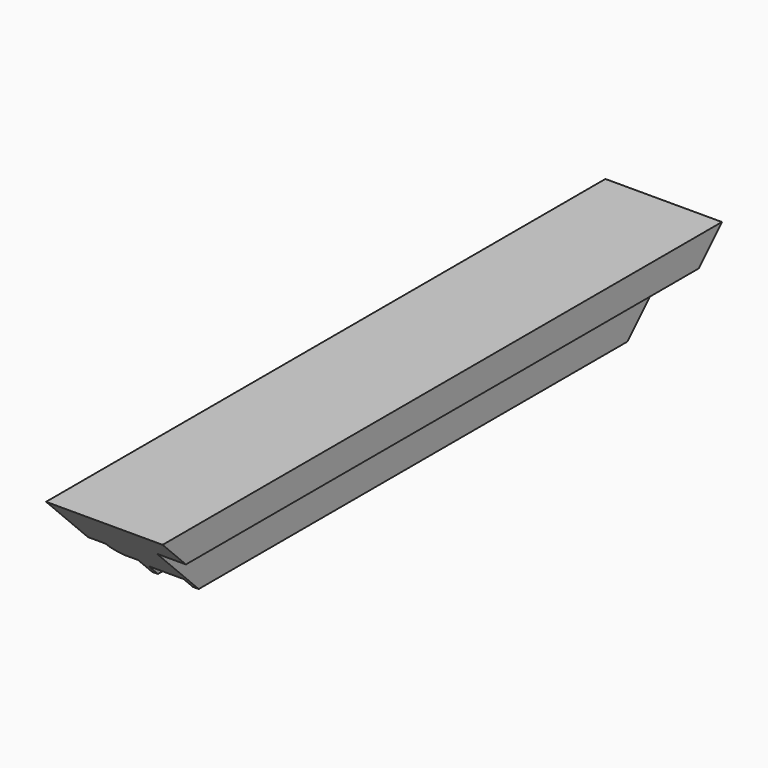
from build123d import *

# Parameters (mm, degrees)
F1_DEPTH = 304.8
F3_DEPTH = 50.8
F4_R     = 5.07999


# Not quite as in the source:
# - a fillet or chamfer is up to 0.001 mm smaller than in the source, because OpenCascade refuses the exact size


with BuildPart() as f1:
    # F0 (on Front) → F1 (new body)
    with BuildSketch(Plane.XZ):
        Polygon((50.8, 0), (0, 0), (0, -22.86), (7.62, -22.86), (7.62, -27.94), (17.78, -27.94), (17.78, -35.56), (20.32, -35.56), (20.32, -30.48), (35.56, -30.48), (35.56, -35.56), (38.1, -35.56), (38.1, -12.7), (50.8, -12.7), align=None)
    extrude(amount=F1_DEPTH)

    # F2 (on face) → F3 (cut)
    with BuildSketch(Plane(origin=(0, 0, 0), x_dir=(0, -1, 0), z_dir=(-1, 0, 0))):
        Polygon((35.56, -35.56), (0, 0), (0, -35.56), align=None)
        Polygon((304.8, -35.56), (304.8, 0), (269.24, -35.56), align=None)
    extrude(amount=-F3_DEPTH, mode=Mode.SUBTRACT)

    # F4 (radius 5.08 in the source; OpenCascade refuses exactly that, so slightly less here)
    f4_edges = [f1.edges().sort_by_distance(p)[0] for p in [
        (7.62, -152.4, -27.94),
    ]]
    fillet(f4_edges, radius=F4_R)


solid = f1.part
